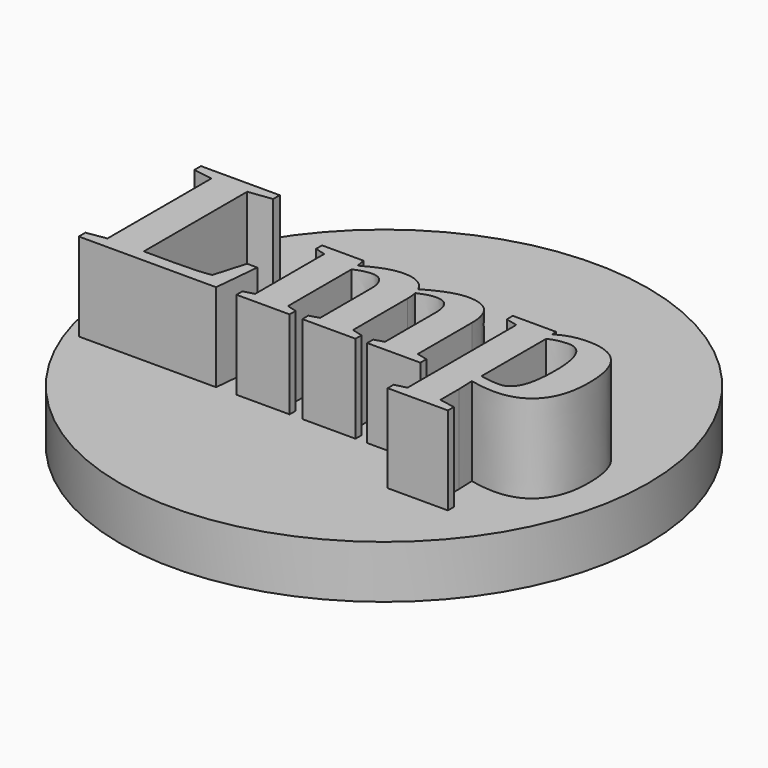
from build123d import *

# Parameters (mm, degrees)
F0_R         = 6
F1_DEPTH     = 1.2
F2_TEXT_SIZE = 5.2932330827
F3_DEPTH     = 2


# Not quite as in the source:
# - Text() gives the source's letters only with a copy of the font that has no kerning and outlines rounded to 1/6400 em; it was checked with that copy


with BuildPart() as f1:
    # F0 (on Top) → F1 (new body)
    with BuildSketch(Plane.XY):
        Circle(F0_R)
    extrude(amount=F1_DEPTH)

    # F2 (on face) → F3 (join)
    with BuildSketch(Plane.XY.offset(1.2)):
        with Locations((-5.5, -1.9055639098)):
            Text('Lmp', F2_TEXT_SIZE, font='Tinos', font_style=FontStyle.BOLD, text_align=(TextAlign.LEFT, TextAlign.BOTTOM))
    extrude(amount=F3_DEPTH)


solid = f1.part
